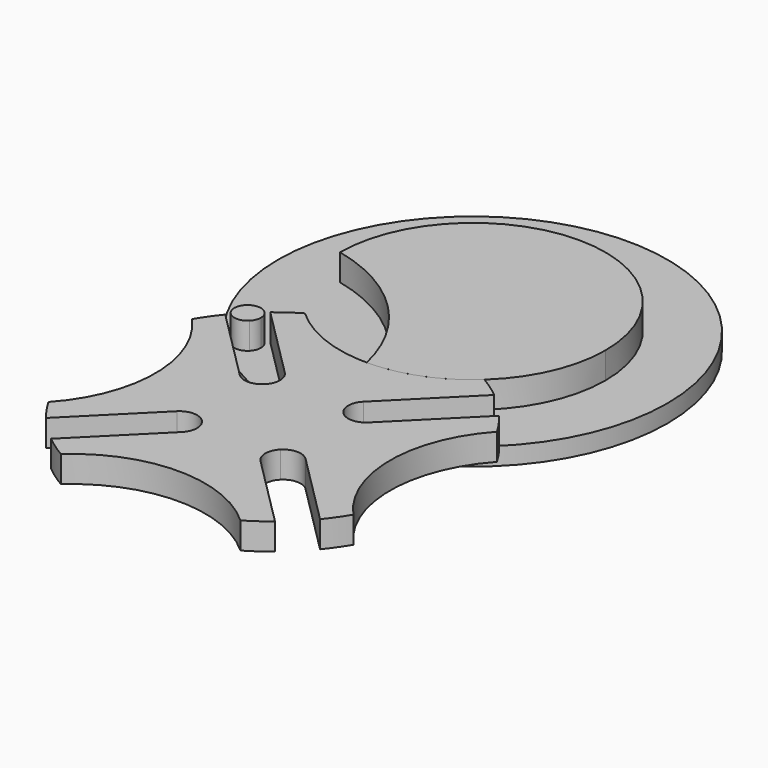
from build123d import *

# Parameters (mm, degrees)
F1_DEPTH    = 3
F2_T1_DEPTH = 3
F3_COUNT    = 4
F4_DEPTH    = 3
F5_R        = 22
F6_DEPTH    = 2
F7_DEPTH    = 3


# Not quite as in the source:
# - a fillet or chamfer that OpenCascade refuses, or shapes differently, is made with other operations: its cross-section is extruded or revolved along the edge and cut away or added


with BuildPart() as f1:
    # F0 (on Top) → F1 (new body)
    with BuildSketch(Plane.XY):
        with BuildLine():
            ThreePointArc((12.6570337171, 15.4854608418), (11.43476766, 16.4087198941), (10.1454269255, 17.2357277914))
            ThreePointArc((10.1454269255, 17.2357277914), (5.443888691, 14.3070012737), (0, 13.2842712475))
            ThreePointArc((0, 13.2842712475), (-5.443888691, 14.3070012737), (-10.1454269255, 17.2357277914))
            ThreePointArc((-10.1454269255, 17.2357277914), (-11.43476766, 16.4087198941), (-12.6570337171, 15.4854608418))
            Line((-12.6570337171, 15.4854608418), (-3.7836501514, 6.6120772761))
            ThreePointArc((-3.7836501514, 6.6120772761), (0, 6.2842712475), (3.7836501514, 6.6120772761))
            Line((3.7836501514, 6.6120772761), (12.6570337171, 15.4854608418))
        make_face()
        with BuildLine():
            Line((3.0294372515, 5.8578643763), (3.7836501514, 6.6120772761))
            ThreePointArc((3.7836501514, 6.6120772761), (0, 6.2842712475), (-3.7836501514, 6.6120772761))
            Line((-3.7836501514, 6.6120772761), (-3.0294372515, 5.8578643763))
            Line((-3.0294372515, 5.8578643763), (-4.4436508139, 4.4436508139))
            Line((-4.4436508139, 4.4436508139), (0, 0))
            Line((0, 0), (4.4436508139, 4.4436508139))
            Line((4.4436508139, 4.4436508139), (3.0294372515, 5.8578643763))
        make_face()
    extrude(amount=F1_DEPTH)

    # F2: fillet of radius 2 on 2 edges, made by hand

    # F2_s2 → F2_t1 (join)
    with BuildSketch(Plane.XY):
        with BuildLine():
            ThreePointArc((-4.4436508139, 7.2720779386), (-3.8578643763, 5.8578643763), (-4.4436508139, 4.4436508139))
            Line((-4.4436508139, 4.4436508139), (-3.0294372515, 5.8578643763))
            Line((-3.0294372515, 5.8578643763), (-4.4436508139, 7.2720779386))
        make_face()
        with BuildLine():
            ThreePointArc((4.4436508139, 4.4436508139), (3.8578643763, 5.8578643763), (4.4436508139, 7.2720779386))
            Line((4.4436508139, 7.2720779386), (3.0294372515, 5.8578643763))
            Line((3.0294372515, 5.8578643763), (4.4436508139, 4.4436508139))
        make_face()
    extrude(amount=F2_T1_DEPTH)

    # F3: F1 ×4 about axis
    f3_axis = Axis((0, 0, 1.5), (0, 0, -1))


with BuildPart() as f1_1:
    add(f1.part)
    for i in range(1, F3_COUNT):
        add(f1.part.rotate(f3_axis, i * 360 / F3_COUNT))


with BuildPart() as f4:
    # F0 (on Top) → F4 (new body)
    with BuildSketch(Plane.XY):
        with BuildLine():
            ThreePointArc((10.1454269255, 17.2357277914), (13.7328329904, 22.2502594759), (15, 28.2842712475))
            ThreePointArc((15, 28.2842712475), (0, 43.2842712475), (-15, 28.2842712475))
            ThreePointArc((-15, 28.2842712475), (-8.079180403, 25.220367714), (-2.7924795837, 19.8040919452))
            ThreePointArc((-2.7924795837, 19.8040919452), (3.8943012543, 19.6171969899), (10.1454269255, 17.2357277914))
        make_face()
    extrude(amount=F4_DEPTH)



with BuildPart() as f4b:
    # F0 (on Top) → F4, piece 2 (new body)
    with BuildSketch(Plane.XY):
        with BuildLine():
            ThreePointArc((-12.6421356237, 14.1421356237), (-12.7457951685, 14.6900711429), (-13.0424467346, 15.162275))
            ThreePointArc((-13.0424467346, 15.162275), (-13.6018583504, 14.6625185222), (-14.1421356237, 14.1421356237))
            Line((-14.1421356237, 14.1421356237), (-13.081475452, 13.081475452))
            ThreePointArc((-13.081475452, 13.081475452), (-12.756316325, 13.5681104752), (-12.6421356237, 14.1421356237))
        make_face()
    extrude(amount=F4_DEPTH)


with BuildPart() as f4_1:
    add(f4.part)

    add(f4b.part)  # F6 merges F4b
    # F5 (on Top) → F6 (join)
    with BuildSketch(Plane.XY):
        with Locations((0, 28.2842712475)):
            Circle(F5_R)
    extrude(amount=-F6_DEPTH)

    # F0 (on Top) → F7 (join)
    with BuildSketch(Plane.XY):
        with BuildLine():
            ThreePointArc((0, 13.2842712475), (5.443888691, 14.3070012737), (10.1454269255, 17.2357277914))
            ThreePointArc((10.1454269255, 17.2357277914), (3.8943012543, 19.6171969899), (-2.7924795837, 19.8040919452))
            ThreePointArc((-2.7924795837, 19.8040919452), (-1.1049131261, 16.6689586115), (0, 13.2842712475))
        make_face()
        with BuildLine():
            ThreePointArc((-14.1421356237, 14.1421356237), (-13.6018583504, 14.6625185222), (-13.0424467346, 15.162275))
            ThreePointArc((-13.0424467346, 15.162275), (-15.2027957955, 15.2027957955), (-15.162275, 13.0424467346))
            ThreePointArc((-15.162275, 13.0424467346), (-14.6625185222, 13.6018583504), (-14.1421356237, 14.1421356237))
        make_face()
        with BuildLine():
            Line((-13.081475452, 13.081475452), (-14.1421356237, 14.1421356237))
            ThreePointArc((-14.1421356237, 14.1421356237), (-14.6625185222, 13.6018583504), (-15.162275, 13.0424467346))
            ThreePointArc((-15.162275, 13.0424467346), (-14.1140056768, 12.6423994116), (-13.081475452, 13.081475452))
        make_face()
    extrude(amount=F7_DEPTH)


solid = Compound([f1_1.part, f4_1.part])
